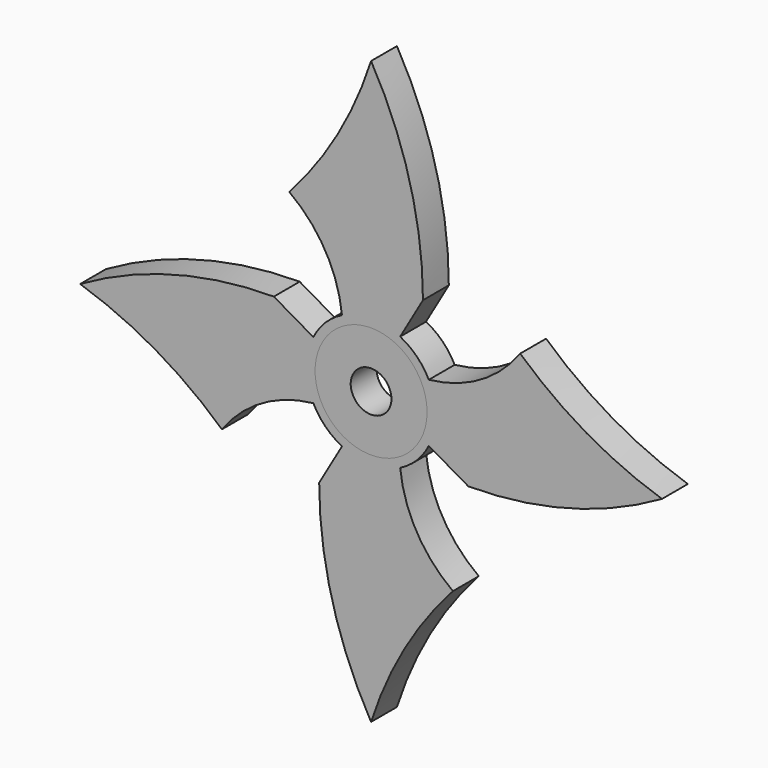
from build123d import *

# Parameters (mm, degrees)
F1_R     = 11
F2_DEPTH = 6.35
F3_COUNT = 4
F4_R     = 11
F4_R_2   = 4
F5_DEPTH = 6.35


with BuildPart() as f2:
    # F1 (on Front) → F2 (new body)
    with BuildSketch(Plane.XZ):
        with BuildLine():
            ThreePointArc((-5.715, 11.3414626482), (-6.6599361859, -10.8136603424), (12.7, 0))
            ThreePointArc((12.7, 0), (10.8136603424, 6.6599361859), (5.715, 11.3414626482))
            ThreePointArc((5.715, 11.3414626482), (0, 12.7), (-5.715, 11.3414626482))
        make_face()
        Circle(F1_R, mode=Mode.SUBTRACT)
        with BuildLine():
            ThreePointArc((-5.715, 11.3414626482), (0, 12.7), (5.715, 11.3414626482))
            Line((5.715, 11.3414626482), (10.1951265992, 19.1012695423))
            ThreePointArc((10.1951265992, 19.1012695423), (7.5986795153, 38.7958068413), (0, 57.15))
            ThreePointArc((0, 57.15), (-6.5543455598, 42.3650839343), (-16.0812856856, 29.2963961415))
            ThreePointArc((-16.0812856856, 29.2963961415), (-8.9828079425, 21.4247485151), (-5.715, 11.3414626482))
        make_face()
    extrude(amount=F2_DEPTH)

    # F3: F2 ×4 about axis
    f3_axis = Axis((0, -6.35, 0), (0, -1, 0))


with BuildPart() as f2_1:
    add(f2.part)
    for i in range(1, F3_COUNT):
        add(f2.part.rotate(f3_axis, i * 360 / F3_COUNT))


with BuildPart() as f5:
    # F4 (on Front) → F5 (new body)
    with BuildSketch(Plane.XZ):
        Circle(F4_R)
        Circle(F4_R_2, mode=Mode.SUBTRACT)
    extrude(amount=F5_DEPTH)


solid = Compound([f2_1.part, f5.part])
